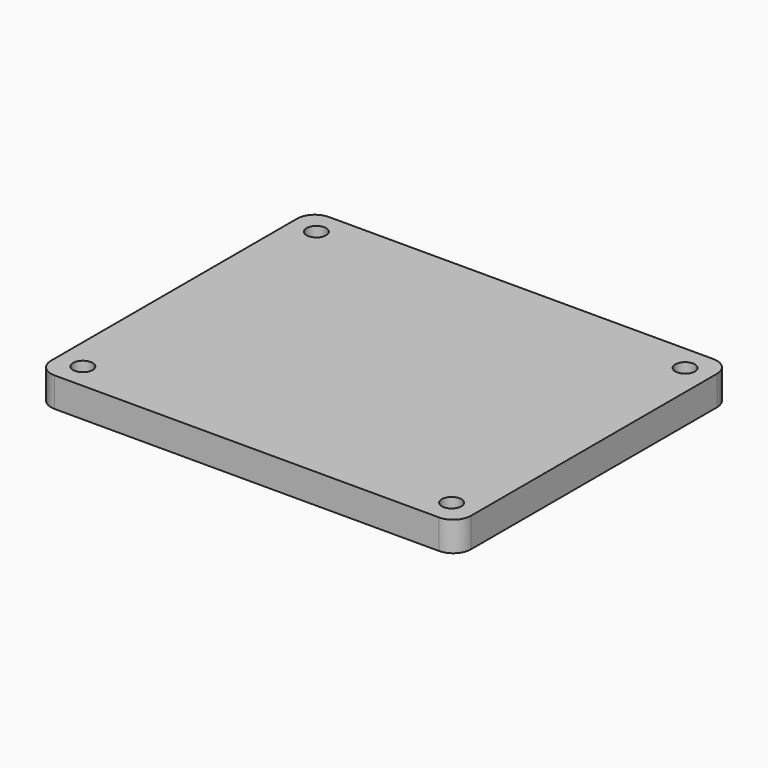
from build123d import *

# Parameters (mm, degrees)
F0_W     = 71
F0_H     = 58
F1_DEPTH = 5.00012
F2_R     = 3
F3_R     = 1.651
F4_DEPTH = 5.00112
F5_R     = 3.556
F5_R_2   = 1.778
F6_DEPTH = 2.5
F8_DEPTH = 3.5


# Not quite as in the source:
# - after a boolean that leaves OpenCascade's solid faulty, fix() repairs it
# - a feature names something its author has since deleted; it is built from what else it names


with BuildPart() as f1:
    # F0 (on Top) → F1 (new body)
    with BuildSketch(Plane.XY):
        Rectangle(F0_W, F0_H)
    extrude(amount=F1_DEPTH)

    # F2
    f2_edges = [f1.edges().sort_by_distance(p)[0] for p in [
        (-35.5, 29, 2.50006),
        (35.5, 29, 2.50006),
        (35.5, -29, 2.50006),
        (-35.5, -29, 2.50006),
    ]]
    fillet(f2_edges, radius=F2_R)

    # F3 (on face) → F4 (cut, through all)
    with BuildSketch(Plane.XY.offset(5.00012)):
        with Locations((-31.1785, 24.6761)):
            Circle(F3_R)
        with Locations((-31.1785, -24.6761)):
            Circle(F3_R)
        with Locations((31.1785, -24.6761)):
            Circle(F3_R)
        with Locations((31.1785, 24.6761)):
            Circle(F3_R)
    extrude(amount=-F4_DEPTH, mode=Mode.SUBTRACT)

    # F5 (on face) → F6 (join)
    with BuildSketch(Plane(origin=(0, 0, 0), x_dir=(1, 0, 0), z_dir=(0, 0, -1))):
        with Locations((-28, 17.875)):
            Circle(F5_R)
        with Locations((-28, 17.875)):
            Circle(F5_R_2, mode=Mode.SUBTRACT)
        with Locations((28, 17.875)):
            Circle(F5_R)
        with Locations((28, 17.875)):
            Circle(F5_R_2, mode=Mode.SUBTRACT)
        with Locations((28, -17.875)):
            Circle(F5_R)
        with Locations((28, -17.875)):
            Circle(F5_R_2, mode=Mode.SUBTRACT)
        with Locations((-28, -17.875)):
            Circle(F5_R)
        with Locations((-28, -17.875)):
            Circle(F5_R_2, mode=Mode.SUBTRACT)
    extrude(amount=F6_DEPTH)

    # F7 (on face) → F8 (cut)
    with BuildSketch(Plane(origin=(0, 0, 0), x_dir=(1, 0, 0), z_dir=(0, 0, -1))):
        with BuildLine():
            ThreePointArc((28, 14.319), (25.4855282861, 15.3605282861), (24.444, 17.875))
            Line((24.444, 17.875), (-24.444, 17.875))
            ThreePointArc((-24.444, 17.875), (-25.4855282861, 15.3605282861), (-28, 14.319))
            Line((-28, 14.319), (-28, -14.319))
            ThreePointArc((-28, -14.319), (-25.4855282861, -15.3605282861), (-24.444, -17.875))
            Line((-24.444, -17.875), (24.444, -17.875))
            ThreePointArc((24.444, -17.875), (25.4855282861, -15.3605282861), (28, -14.319))
            Line((28, -14.319), (28, 14.319))
        make_face()
    extrude(amount=-F8_DEPTH, mode=Mode.SUBTRACT)

    add(f1.part.fix(), mode=Mode.REPLACE)


solid = f1.part
